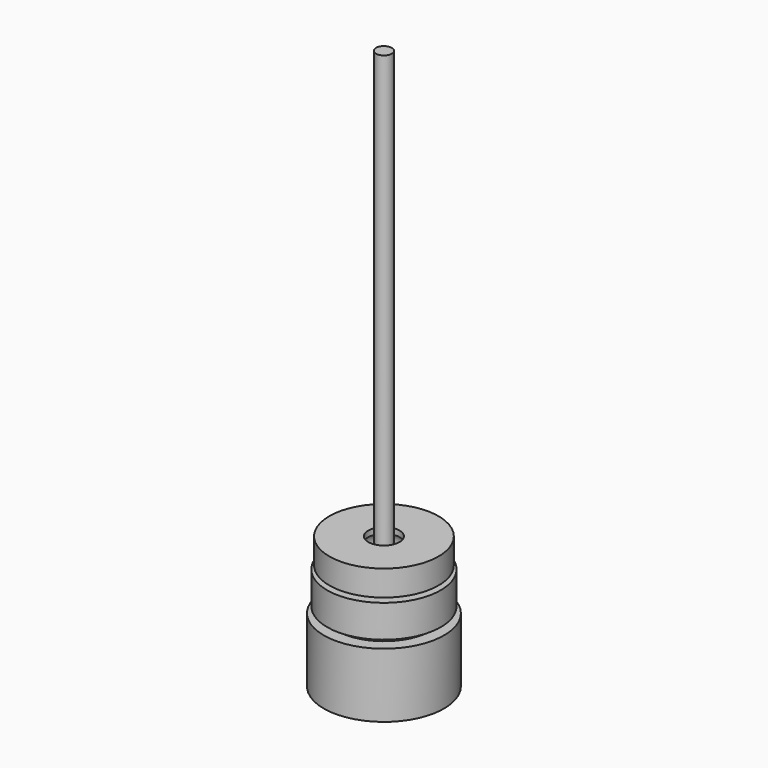
from build123d import *


# Not quite as in the source:
# - the program builds the solid bodies; features that only make, move or delete a surface that nothing else refers to are left out


with BuildPart() as f1:
    # F0 (on Front) → F1 (revolve)
    with BuildSketch(Plane.XZ):
        with BuildLine():
            ThreePointArc((0, -7), (-4.9497474683, -4.9497474683), (-7, 0))
            ThreePointArc((-7, 0), (-14.7014178909, 6.197156881), (-17.9689702317, 15.5266634402))
            Line((-17.9689702317, 15.5266634402), (-22.7487955556, 15.5266634402))
            Line((-22.7487955556, 15.5266634402), (-22.7487955556, -8.8577289134))
            Line((-22.7487955556, -8.8577289134), (0, -8.8577289134))
            Line((0, -8.8577289134), (0, -7))
        make_face()
    revolve(axis=Axis((0, 0, 1.4671878889), (0, 0, -1)))


with BuildPart() as f5:
    # F4 (on Front) → F5 (revolve)
    with BuildSketch(Plane.XZ):
        with BuildLine():
            Line((0, 202.8778705808), (-3, 202.8778705808))
            Line((-3, 202.8778705808), (-3, -2.5413907133))
            ThreePointArc((-3, -2.5413907133), (-2.1464811113, -4.8387767003), (0, -6.0216104612))
            Line((0, -6.0216104612), (0, 202.8778705808))
        make_face()
    revolve(axis=Axis((0, 0, 98.4281300598), (0, 0, -1)))


with BuildPart() as f7:
    # F6 (on Front) → F7 (revolve)
    with BuildSketch(Plane.XZ):
        with BuildLine():
            ThreePointArc((-7.5039273792, 19.902308523), (-13.269900953, 23.6491971564), (-15.5229725728, 30.1460651681))
            Line((-15.5229725728, 30.1460651681), (-21.4822479671, 30.1460651681))
            Line((-21.4822479671, 30.1460651681), (-21.4822479671, 17.8516013548))
            Line((-21.4822479671, 17.8516013548), (-7.3899991428, 17.8516013548))
            Line((-7.3899991428, 17.8516013548), (-7.5039273792, 19.902308523))
        make_face()
    revolve(axis=Axis((0, 0, 30.2875973284), (0, 0, -1)))


with BuildPart() as f9:
    # F8 (on Front) → F9 (revolve)
    with BuildSketch(Plane.XZ):
        with BuildLine():
            ThreePointArc((-11.0752568096, 31.4721912146), (-10.0988489164, 36.3099864549), (-5.9177334867, 38.9321818948))
            Line((-5.9177334867, 38.9321818948), (-5.9177334867, 41.1425493658))
            Line((-5.9177334867, 41.1425493658), (-20.655285567, 41.1425493658))
            Line((-20.655285567, 41.1425493658), (-20.655285567, 31.4721912146))
            Line((-20.655285567, 31.4721912146), (-11.0752568096, 31.4721912146))
        make_face()
    revolve(axis=Axis((0, 0, 38.9782302082), (0, 0, -1)))


solid = Compound([f1.part, f5.part, f7.part, f9.part])
